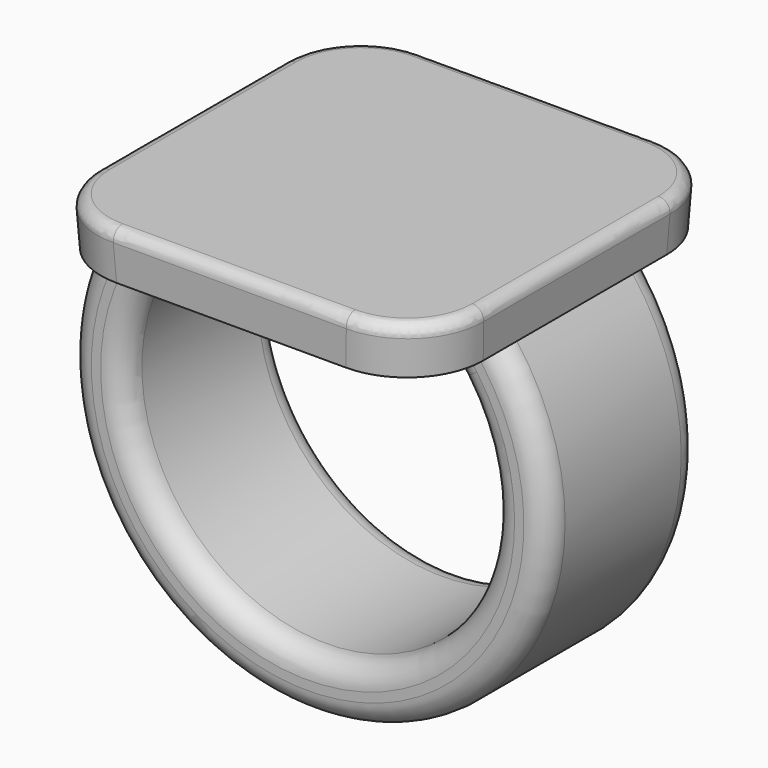
from build123d import *

# Parameters (mm, degrees)
F0_W          = 25.4
F0_H          = 25.4
F1_DEPTH      = 3.175
F1_TAPER      = -3
F3_W          = 5.08
F3_H          = 12.7
F6_DEPTH      = 6.35
F6_DEPTH_BACK = 6.35
F7_R          = 5.08
F8_R          = 1.524
F9_R          = 0.762


with BuildPart() as f1:
    # F0 (on Top) → F1 (new body)
    with BuildSketch(Plane.XY):
        Rectangle(F0_W, F0_H)
    extrude(amount=F1_DEPTH, taper=F1_TAPER)

    # F4: sweep along a path in F2
    with BuildLine(Plane.XZ) as f4_path:
        ThreePointArc((-10.16, 0), (0, -23.5582897328), (10.16, 0))
    # F3 (on face) → F4 (sweep)
    with BuildSketch(Plane(origin=(0, 0, 0), x_dir=(1, 0, 0), z_dir=(0, 0, -1))):
        with Locations((-10.16, 0)):
            Rectangle(F3_W, F3_H)
    sweep(path=f4_path.line)

    # F5 (on Front) → F6 (join, two sides)
    with BuildSketch(Plane.XZ) as f6_sk:
        with BuildLine():
            ThreePointArc((7.62, 0), (8.9072265211, -1.1822790439), (10.0130578512, -2.535746045))
            Line((10.0130578512, -2.535746045), (10.16, 0))
            Line((10.16, 0), (7.62, 0))
        make_face()
    extrude(amount=F6_DEPTH)
    extrude(f6_sk.sketch, amount=-F6_DEPTH_BACK)

    # F7
    f7_edges = [f1.edges().sort_by_distance(p)[0] for p in [
        (-12.783197, -12.783197, 1.5875),
        (-12.783197, 12.783197, 1.5875),
        (12.783197, 12.783197, 1.5875),
        (12.783197, -12.783197, 1.5875),
    ]]
    fillet(f7_edges, radius=F7_R)

    # F8
    f8_edges = [f1.edges().sort_by_distance(p)[0] for p in [
        (-1.743325, -6.35, -21.711017),
        (-1.743325, 6.35, -21.711017),
        (8.907227, 6.35, -1.182279),
        (0, 6.35, -25.501344),
        (8.907227, -6.35, -1.182279),
        (0, -6.35, -25.501344),
    ]]
    fillet(f8_edges, radius=F8_R)

    # F9
    f9_edges = [f1.edges().sort_by_distance(p)[0] for p in [
        (0, 12.866395, 3.175),
        (11.381378, 11.381378, 3.175),
        (-11.381378, 11.381378, 3.175),
        (12.866395, 0, 3.175),
        (-12.866395, 0, 3.175),
        (11.381378, -11.381378, 3.175),
        (-11.381378, -11.381378, 3.175),
        (0, -12.866395, 3.175),
    ]]
    fillet(f9_edges, radius=F9_R)


solid = f1.part
